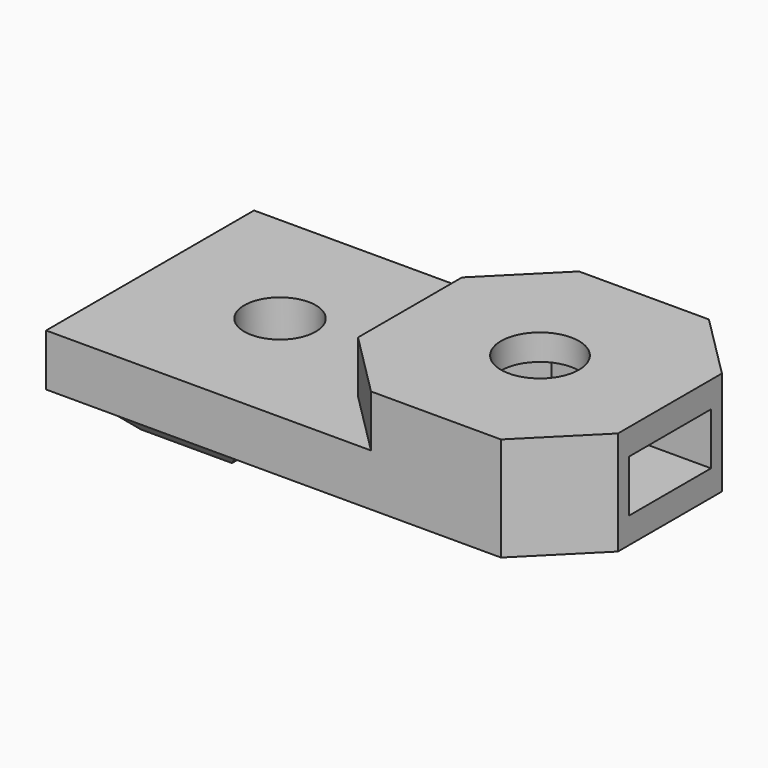
from build123d import *

# Parameters (mm, degrees)
F0_W      = 40
F0_H      = 20
F1_DEPTH  = 4
F2_W      = 20
F2_H      = 20
F3_DEPTH  = 4
F4_W      = 9
F4_H      = 20
F5_DEPTH  = 1
F6_SIZE   = 0.99999
F7_R      = 2.75
F8_DEPTH  = 5.001
F9_SIZE   = 5
F10_R     = 3
F11_DEPTH = 9.001
F13_DEPTH = 2


# Not quite as in the source:
# - a fillet or chamfer is up to 0.001 mm smaller than in the source, because OpenCascade refuses the exact size


with BuildPart() as f1:
    # F0 (on Top) → F1 (new body)
    with BuildSketch(Plane.XY):
        with Locations((20, 10)):
            Rectangle(F0_W, F0_H)
    extrude(amount=F1_DEPTH)

    # F2 (on face) → F3 (join)
    with BuildSketch(Plane.XY.offset(4)):
        with Locations((30, 10)):
            Rectangle(F2_W, F2_H)
    extrude(amount=F3_DEPTH)

    # F4 (on face) → F5 (join)
    with BuildSketch(Plane(origin=(0, 0, 0), x_dir=(1, 0, 0), z_dir=(0, 0, -1))):
        with Locations((10, -10)):
            Rectangle(F4_W, F4_H)
    extrude(amount=F5_DEPTH)

    # F6 (size 1 in the source; OpenCascade refuses exactly that, so slightly less here)
    f6_edges = [f1.edges().sort_by_distance(p)[0] for p in [
        (10, 0, -1),
        (5.5, 10, -1),
        (10, 20, -1),
        (14.5, 10, -1),
    ]]
    chamfer(f6_edges, length=F6_SIZE)

    # F7 (on face) → F8 (cut, through all)
    with BuildSketch(Plane.XY.offset(4)):
        with Locations((10, 10)):
            Circle(F7_R)
    extrude(amount=-F8_DEPTH, mode=Mode.SUBTRACT)

    # F9
    f9_edges = [f1.edges().sort_by_distance(p)[0] for p in [
        (40, 0, 4),
        (40, 20, 4),
        (20, 0, 6),
        (20, 20, 6),
    ]]
    chamfer(f9_edges, length=F9_SIZE)

    # F10 (on face) → F11 (cut, through all)
    with BuildSketch(Plane.XY.offset(8)):
        with Locations((30, 10)):
            Circle(F10_R)
    extrude(amount=-F11_DEPTH, mode=Mode.SUBTRACT)

    # F12 (on face) → F13 (cut, symmetric)
    with BuildSketch(Plane.XY.offset(4)):
        Polygon((25.4389328734, 10), (27.7194664367, 6.05), (40, 6.05), (40, 13.95), (27.7194664367, 13.95), align=None)
    extrude(amount=F13_DEPTH, both=True, mode=Mode.SUBTRACT)


solid = f1.part
